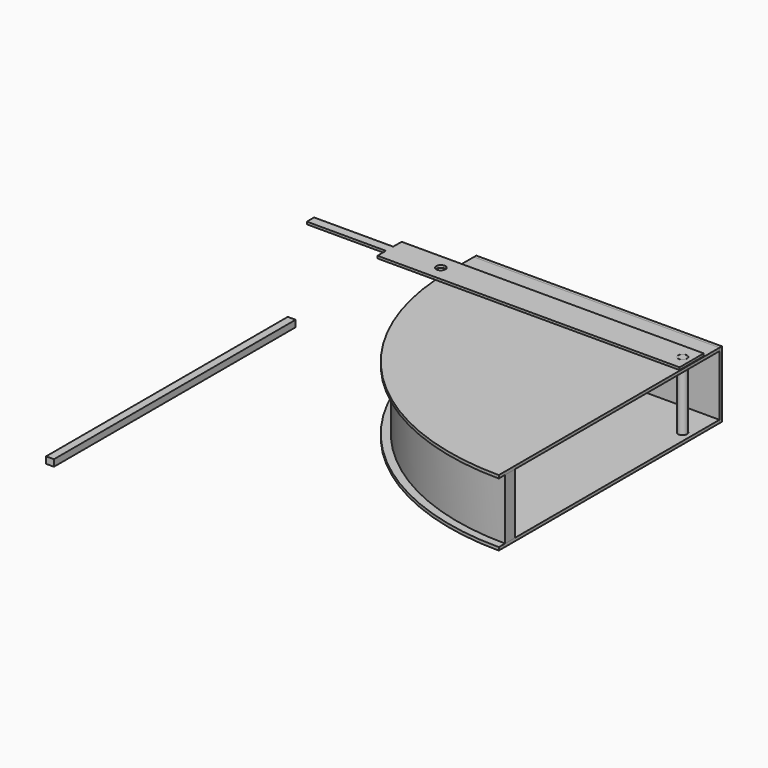
from build123d import *

# Parameters (mm, degrees)
F1_DEPTH  = 100
F4_DEPTH  = 5
F6_W      = 393.5
F6_H      = 50
F6_W_2    = 13
F7_DEPTH  = 5
F9_W      = 406.5
F9_H      = 110
F10_DEPTH = 5.1
F11_R     = 7.5
F12_DEPTH = 110.001
F14_R     = 7.25
F15_DEPTH = 120
F17_R     = 7.5
F17_W     = 130.9452056885
F17_H     = 15
F18_DEPTH = 4
F0_W      = 20
F0_H      = 50
F19_DEPTH = 100
F21_W     = 13
F21_H     = 500
F22_DEPTH = 11


# Not quite as in the source:
# - a feature names something its author has since deleted; it is built from what else it names
# - the program builds the solid bodies; features that only make, move or delete a surface that nothing else refers to are left out


with BuildPart() as f1:
    # F0 (on Top) → F1 (new body)
    with BuildSketch(Plane.XY):
        with BuildLine():
            ThreePointArc((0, -373.5), (-264.1043827732, -264.1043827732), (-373.5, 0))
            Line((-373.5, 0), (-393.5, 0))
            ThreePointArc((-393.5, 0), (-278.2465183969, -278.2465183969), (0, -393.5))
            Line((0, -393.5), (0, -373.5))
        make_face()
    extrude(amount=F1_DEPTH)


with BuildPart() as f4:
    # F3 (on offset) → F4 (new body)
    with BuildSketch(Plane(origin=(0, 0, 0), x_dir=(1, 0, 0), z_dir=(0, 0, -1))):
        with BuildLine():
            Line((-393.5, 0), (0, 0))
            Line((0, 0), (0, 393.5))
            ThreePointArc((0, 393.5), (-278.2465183969, 278.2465183969), (-393.5, 0))
        make_face()
        Polygon((0, -50), (0, 0), (-393.5, 0), (-406.5, 0), (-406.5, -50), align=None)
        with BuildLine():
            ThreePointArc((-393.5, 0), (-278.2465183969, 278.2465183969), (0, 393.5))
            Line((0, 393.5), (0, 406.5))
            ThreePointArc((0, 406.5), (-287.4389065523, 287.4389065523), (-406.5, 0))
            Line((-406.5, 0), (-393.5, 0))
        make_face()
    extrude(amount=F4_DEPTH)


with BuildPart() as f7:
    # F6 (on offset) → F7 (new body)
    with BuildSketch(Plane.XY.offset(100)):
        with BuildLine():
            Line((0, -393.5), (0, 0))
            Line((0, 0), (-393.5, 0))
            ThreePointArc((-393.5, 0), (-278.2465183969, -278.2465183969), (0, -393.5))
        make_face()
        with Locations((-196.75, 25)):
            Rectangle(F6_W, F6_H)
        with BuildLine():
            Line((0, -406.5), (0, -393.5))
            ThreePointArc((0, -393.5), (-278.2465183969, -278.2465183969), (-393.5, 0))
            Line((-393.5, 0), (-406.5, 0))
            ThreePointArc((-406.5, 0), (-287.4389065523, -287.4389065523), (0, -406.5))
        make_face()
        with Locations((-400, 25)):
            Rectangle(F6_W_2, F6_H)
    extrude(amount=F7_DEPTH)


with BuildPart() as f10:
    # F9 (on offset) → F10 (new body)
    with BuildSketch(Plane(origin=(0, 50, 0), x_dir=(-1, 0, 0), z_dir=(0, 1, 0))):
        with Locations((203.25, 50)):
            Rectangle(F9_W, F9_H)
    extrude(amount=F10_DEPTH)


with BuildPart() as f12_tool:
    # F11 (on face) → F12 (new body, through all)
    with BuildSketch(Plane.XY.offset(105)):
        with Locations((-15, -7.5)):
            Circle(F11_R)
    extrude(amount=-F12_DEPTH)


with BuildPart() as f4_1:
    add(f4.part)

    # F12: cut by f12_tool
    add(f12_tool.part, mode=Mode.SUBTRACT)


with BuildPart() as f7_1:
    add(f7.part)

    # F12: cut by f12_tool
    add(f12_tool.part, mode=Mode.SUBTRACT)


with BuildPart() as f15:
    # F14 (on offset) → F15 (new body)
    with BuildSketch(Plane.XY.offset(110)):
        with Locations((-15, -7.5)):
            Circle(F14_R)
    extrude(amount=-F15_DEPTH)


with BuildPart() as f18:
    # F17 (on offset) → F18 (new body)
    with BuildSketch(Plane.XY.offset(110)):
        Polygon((-500, -32.5), (0, -32.5), (0, 17.5), (-500, 17.5), (-500, 0), (-500, -15), align=None)
        with Locations((-415, -7.5)):
            Circle(F17_R, mode=Mode.SUBTRACT)
        with Locations((-15, -7.5)):
            Circle(F17_R, mode=Mode.SUBTRACT)
        with Locations((-565.4726028442, -7.5)):
            Rectangle(F17_W, F17_H)
    extrude(amount=-F18_DEPTH)


with BuildPart() as f19:
    # F0 (on Top) → F19 (new body)
    with BuildSketch(Plane.XY):
        with Locations((-383.5, 25)):
            Rectangle(F0_W, F0_H)
    extrude(amount=F19_DEPTH)


with BuildPart() as f22:
    # F21 (on Top) → F22 (new body)
    with BuildSketch(Plane.XY):
        with Locations((-595.9782657623, -340.0288820267)):
            Rectangle(F21_W, F21_H)
    extrude(amount=F22_DEPTH)


solid = Compound([f1.part, f10.part, f4_1.part, f7_1.part, f15.part, f18.part, f19.part, f22.part])
